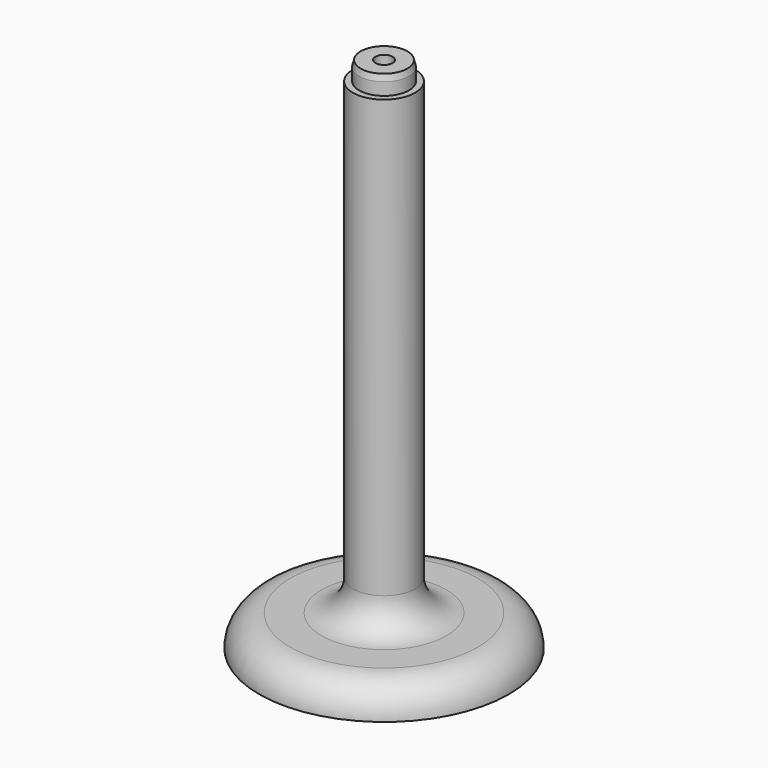
from build123d import *

# Parameters (mm, degrees)
F0_R     = 20
F1_DEPTH = 5
F2_R     = 5
F3_DEPTH = 75
F4_R     = 4
F5_DEPTH = 3
F6_SIZE2 = 1
F6_SIZE  = 0.25
F7_R     = 4.99999
F9_D     = 2.75
F9_DEPTH = 7
F9_TIP   = 0.8261833512


# Not quite as in the source:
# - a fillet or chamfer is up to 0.001 mm smaller than in the source, because OpenCascade refuses the exact size


with BuildPart() as f1:
    # F0 (on Top) → F1 (new body)
    with BuildSketch(Plane.XY):
        Circle(F0_R)
    extrude(amount=F1_DEPTH)

    # F2 (on face) → F3 (join)
    with BuildSketch(Plane.XY.offset(5)):
        Circle(F2_R)
    extrude(amount=F3_DEPTH)

    # F4 (on face) → F5 (join)
    with BuildSketch(Plane.XY.offset(80)):
        Circle(F4_R)
    extrude(amount=F5_DEPTH)

    # F6
    f6_edges = [f1.edges().sort_by_distance(p)[0] for p in [
        (-4, 0, 83),
    ]]
    f6_side = f1.faces().sort_by_distance((0, 0, 83))[0]
    chamfer(f6_edges, length=F6_SIZE, length2=F6_SIZE2, reference=f6_side)

    # F7 (radius 5 in the source; OpenCascade refuses exactly that, so slightly less here)
    f7_edges = [f1.edges().sort_by_distance(p)[0] for p in [
        (-20, 0, 5),
        (-5, 0, 5),
    ]]
    fillet(f7_edges, radius=F7_R)

    # F9
    with Locations(Plane.XY.offset(83)):
        with Locations((0, 0)):
            Hole(F9_D / 2, depth=F9_DEPTH)
            with Locations((0, 0, -(F9_DEPTH + F9_TIP / 2))):  # 118° drill point
                Cone(0, F9_D / 2, F9_TIP, mode=Mode.SUBTRACT)


solid = f1.part
